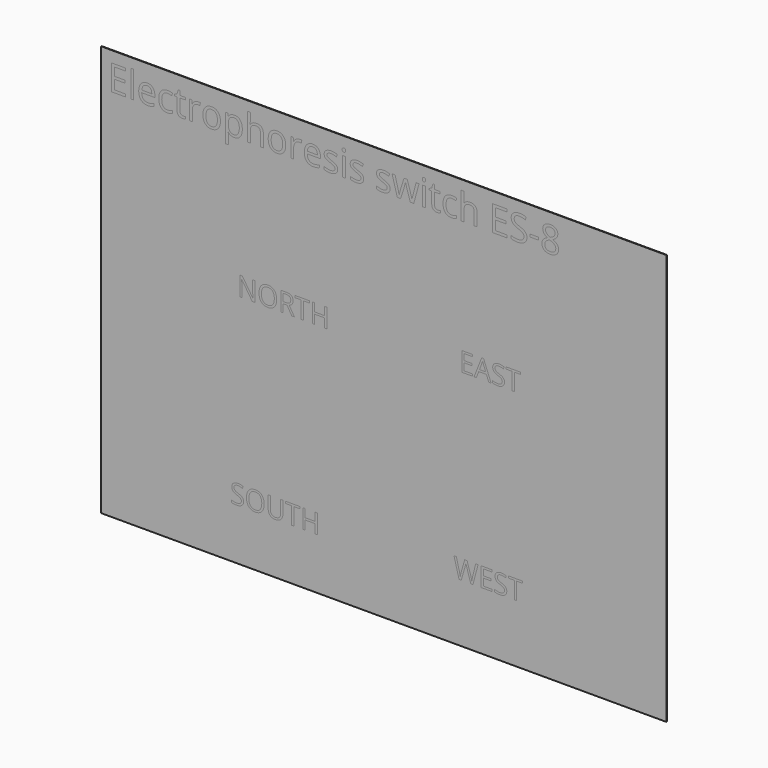
from build123d import *

# Parameters (mm, degrees)
F0_W         = 139.7
F0_H         = 101.6
F1_DEPTH     = 0.127
F2_TEXT_SIZE = 6.6322222222
F3_TEXT_SIZE = 8.8194444444
F4_DEPTH     = 0.127


# Not quite as in the source:
# - Text() gives the source's letters only with a copy of the font that has no kerning and outlines rounded to 1/6400 em; it was checked with that copy


with BuildPart() as f1:
    # F0 (on Front) → F1 (new body)
    with BuildSketch(Plane.XZ):
        Rectangle(F0_W, F0_H)
    extrude(amount=F1_DEPTH)


with BuildPart() as f4:
    # F2 (on Front) + F3 (on Front) → F4 (new body)
    with BuildSketch(Plane.XZ):
        with Locations((-36.2449385389, 7.4277353421)):
            Text('NORTH', F2_TEXT_SIZE, font='Open Sans', text_align=(TextAlign.LEFT, TextAlign.BOTTOM))
        with Locations((18.636027749, 8.8560460527)):
            Text('EAST', F2_TEXT_SIZE, font='Open Sans', text_align=(TextAlign.LEFT, TextAlign.BOTTOM))
        with Locations((-37.9824941161, -38.1209179368)):
            Text('SOUTH', F2_TEXT_SIZE, font='Open Sans', text_align=(TextAlign.LEFT, TextAlign.BOTTOM))
        with Locations((17.2577920946, -36.4449321832)):
            Text('WEST', F2_TEXT_SIZE, font='Open Sans', text_align=(TextAlign.LEFT, TextAlign.BOTTOM))
    with BuildSketch(Plane.XZ):
        with Locations((-68.2146002166, 41.7247582884)):
            Text('Electrophoresis switch ES-8', F3_TEXT_SIZE, font='Open Sans', text_align=(TextAlign.LEFT, TextAlign.BOTTOM))
    extrude(amount=F4_DEPTH)


solid = Compound([f1.part, f4.part])
